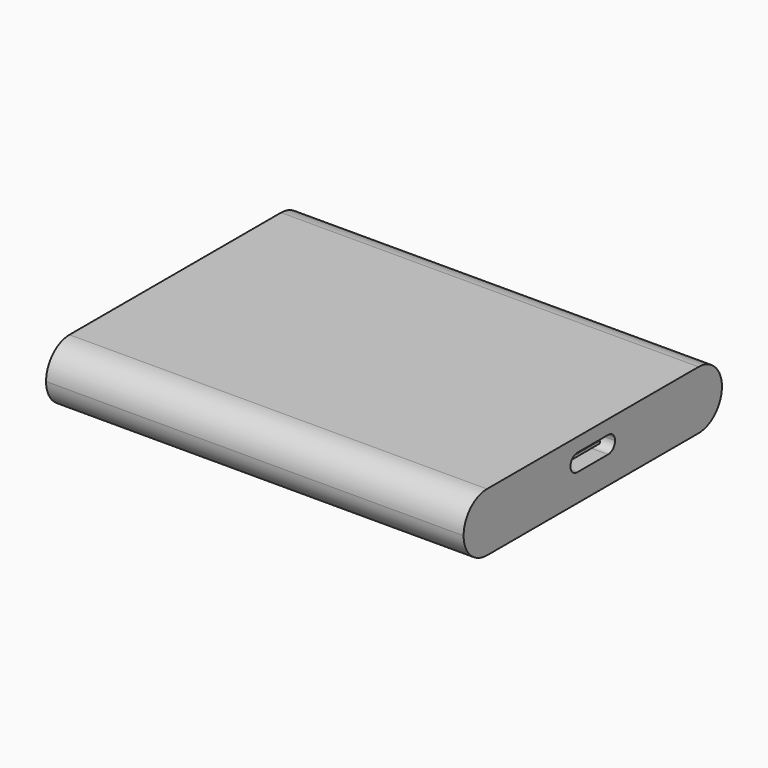
from build123d import *

# Parameters (mm, degrees)
F0_W     = 75
F0_H     = 58
F1_DEPTH = 10.5
F3_R     = 5.24999
F4_DEPTH = 6
F5_W     = 6.9
F5_H     = 0.25
F6_DEPTH = 4.572
F7_R     = 0.24999


# Not quite as in the source:
# - a fillet or chamfer is up to 0.001 mm smaller than in the source, because OpenCascade refuses the exact size


with BuildPart() as f1:
    # F0 (on Top) → F1 (new body)
    with BuildSketch(Plane.XY):
        with Locations((-17.9516240954, -13.4977242947)):
            Rectangle(F0_W, F0_H)
    extrude(amount=F1_DEPTH)

    # F3 (radius 5.25 in the source; OpenCascade refuses exactly that, so slightly less here)
    f3_edges = [f1.edges().sort_by_distance(p)[0] for p in [
        (-17.951624, -42.497724, 10.5),
        (-17.951624, -42.497724, 0),
        (-17.951624, 15.502276, 10.5),
        (-17.951624, 15.502276, 0),
    ]]
    fillet(f3_edges, radius=F3_R)

    # F2 (on face) → F4 (cut)
    with BuildSketch(Plane.YZ.offset(19.5483759046)):
        with BuildLine():
            Line((-10.0477242947, 8), (-13.4977242947, 8))
            Line((-13.4977242947, 8), (-16.9477242947, 8))
            ThreePointArc((-16.9477242947, 8), (-15.8517087838, 7.5460155108), (-15.3977242947, 6.45))
            ThreePointArc((-15.3977242947, 6.45), (-15.8517087838, 5.3539844892), (-16.9477242947, 4.9))
            Line((-16.9477242947, 4.9), (-10.0477242947, 4.9))
            ThreePointArc((-10.0477242947, 4.9), (-11.5977242947, 6.45), (-10.0477242947, 8))
        make_face()
        with BuildLine():
            Line((-10.0477242947, 4.9), (-10.0477242947, 8))
            ThreePointArc((-10.0477242947, 8), (-11.5977242947, 6.45), (-10.0477242947, 4.9))
        make_face()
        with BuildLine():
            ThreePointArc((-8.4977242947, 6.45), (-8.9517087838, 7.5460155108), (-10.0477242947, 8))
            Line((-10.0477242947, 8), (-10.0477242947, 4.9))
            ThreePointArc((-10.0477242947, 4.9), (-8.9517087838, 5.3539844892), (-8.4977242947, 6.45))
        make_face()
        with BuildLine():
            ThreePointArc((-15.3977242947, 6.45), (-15.8517087838, 7.5460155108), (-16.9477242947, 8))
            Line((-16.9477242947, 8), (-16.9477242947, 4.9))
            ThreePointArc((-16.9477242947, 4.9), (-15.8517087838, 5.3539844892), (-15.3977242947, 6.45))
        make_face()
        with BuildLine():
            Line((-16.9477242947, 4.9), (-16.9477242947, 8))
            ThreePointArc((-16.9477242947, 8), (-18.0437398055, 7.5460155108), (-18.4977242947, 6.45))
            ThreePointArc((-18.4977242947, 6.45), (-18.0437398055, 5.3539844892), (-16.9477242947, 4.9))
        make_face()
    extrude(amount=-F4_DEPTH, mode=Mode.SUBTRACT)

    # F5 (on face) → F6 (join)
    with BuildSketch(Plane.YZ.offset(13.5483759046)):
        with Locations((-13.4977242947, 6.575)):
            Rectangle(F5_W, F5_H)
        with Locations((-13.4977242947, 6.325)):
            Rectangle(F5_W, F5_H)
    extrude(amount=F6_DEPTH)

    # F7 (radius 0.25 in the source; OpenCascade refuses exactly that, so slightly less here)
    f7_edges = [f1.edges().sort_by_distance(p)[0] for p in [
        (15.834376, -10.047724, 6.7),
        (15.834376, -10.047724, 6.2),
        (15.834376, -16.947724, 6.7),
        (15.834376, -16.947724, 6.2),
    ]]
    fillet(f7_edges, radius=F7_R)


solid = f1.part
